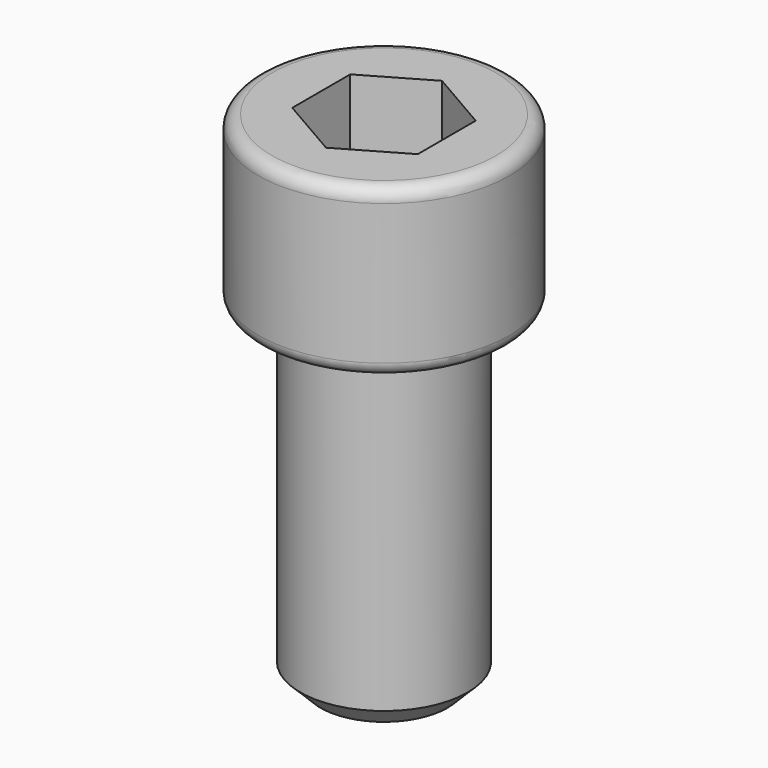
from build123d import *

# Parameters (mm, degrees)
F1_R     = 4.7625
F4_DEPTH = 6.35
F6_DEPTH = 4.826
F2_R     = 3.175
F7_DEPTH = 12.7
F9_SIZE2 = 0.762
F9_SIZE  = 0.762
F10_R    = 0.508


# Not quite as in the source:
# - the program builds the solid bodies; features that only make, move or delete a surface that nothing else refers to are left out


with BuildPart() as f4:
    # F1 (on Top) → F4 (new body)
    with BuildSketch(Plane.XY):
        Circle(F1_R)
    extrude(amount=F4_DEPTH)

    # F5 (on face) → F6 (cut)
    with BuildSketch(Plane.XY.offset(6.35)):
        Polygon((2.38125, -1.3748153285), (2.38125, 1.3748153285), (0, 2.749630657), (-2.38125, 1.3748153285), (-2.38125, -1.3748153285), (0, -2.749630657), align=None)
    extrude(amount=-F6_DEPTH, mode=Mode.SUBTRACT)

    # F2 (on Top) → F7 (join)
    with BuildSketch(Plane.XY):
        Circle(F2_R)
    extrude(amount=-F7_DEPTH)

    # F9
    f9_edges = [f4.edges().sort_by_distance(p)[0] for p in [
        (-3.175, 0, -12.7),
    ]]
    chamfer(f9_edges, length=F9_SIZE, length2=F9_SIZE2)

    # F10
    f10_edges = [f4.edges().sort_by_distance(p)[0] for p in [
        (-4.7625, 0, 6.35),
        (-4.7625, 0, 0),
    ]]
    fillet(f10_edges, radius=F10_R)


solid = f4.part
